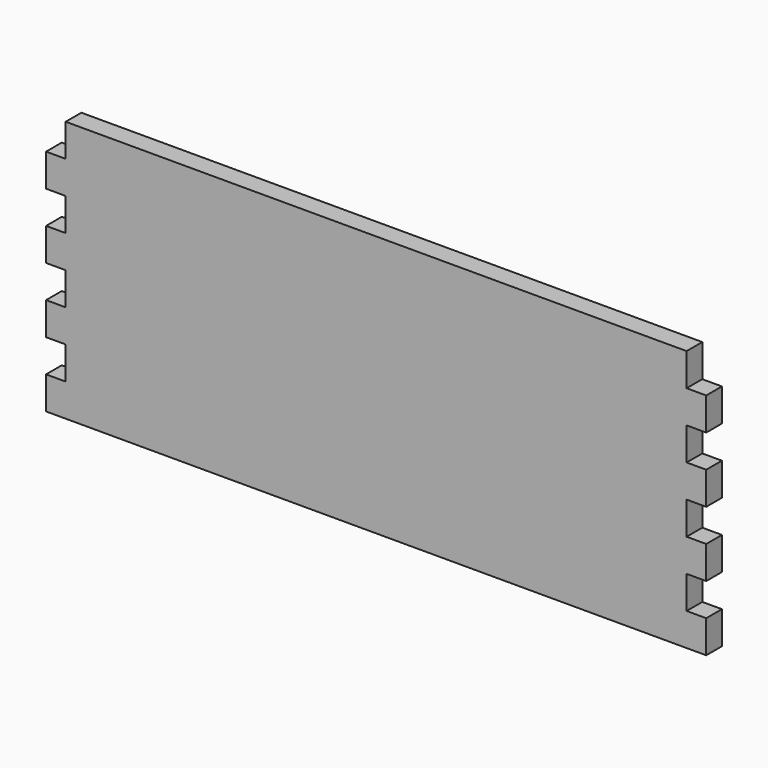
from build123d import *

# Parameters (mm, degrees)
F0_W     = 95
F0_H     = 40
F1_DEPTH = 3
F2_W     = 3
F2_H     = 5
F3_DEPTH = 3


# Not quite as in the source:
# - a feature names something its author has since deleted; it is built from what else it names


with BuildPart() as f1:
    # F0 (on Front) → F1 (new body)
    with BuildSketch(Plane.XZ):
        Rectangle(F0_W, F0_H)
    extrude(amount=F1_DEPTH)

    # F2 (on face) → F3 (join)
    with BuildSketch(Plane.XZ.offset(3)):
        with Locations((-49, -17.5)):
            Rectangle(F2_W, F2_H)
        with Locations((-49, -7.5)):
            Rectangle(F2_W, F2_H)
        with Locations((-49, 2.5)):
            Rectangle(F2_W, F2_H)
        with Locations((-49, 12.5)):
            Rectangle(F2_W, F2_H)
        with Locations((49, -7.5)):
            Rectangle(F2_W, F2_H)
        with Locations((49, -17.5)):
            Rectangle(F2_W, F2_H)
        with Locations((49, 12.5)):
            Rectangle(F2_W, F2_H)
        with Locations((49, 2.5)):
            Rectangle(F2_W, F2_H)
    extrude(amount=-F3_DEPTH)


solid = f1.part
